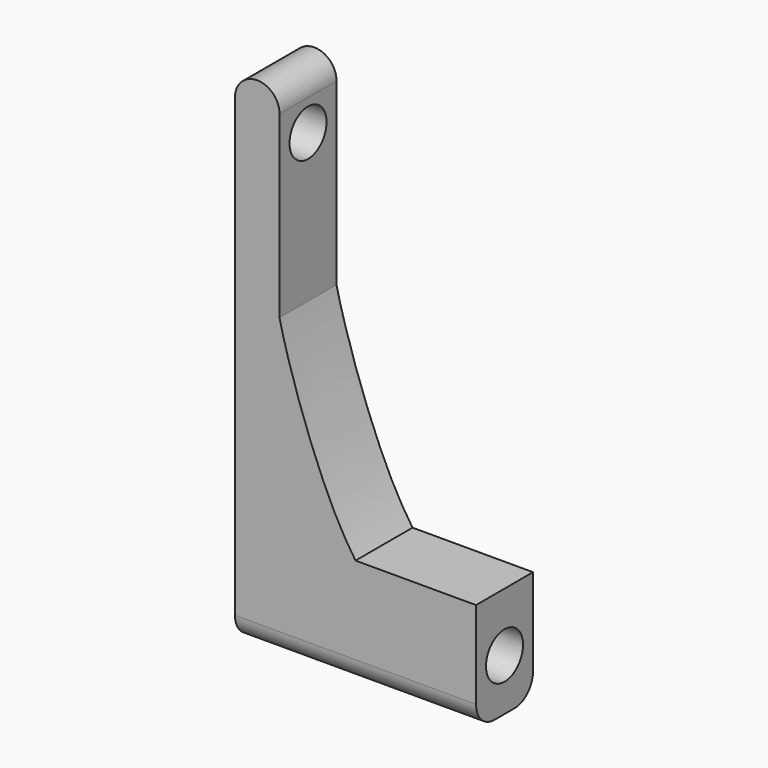
from build123d import *

# Parameters (mm, degrees)
F1_DEPTH = 5.08
F2_R     = 1.651
F4_D     = 3.3


with BuildPart() as f1:
    # F0 (on Front) → F1 (new body)
    with BuildSketch(Plane.XZ):
        with BuildLine():
            Line((-26.6248177087, 44.2240222495), (-26.6248177087, 37.1401777957))
            Line((-26.6248177087, 37.1401777957), (-26.6248177087, 15.790813717))
            Line((-26.6248177087, 15.790813717), (-18.0322819572, 15.790813717))
            Line((-18.0322819572, 15.790813717), (-9.4473101199, 15.790813717))
            Line((-9.4473101199, 15.790813717), (-9.4473101199, 23.6617988805))
            Line((-9.4473101199, 23.6617988805), (-16.3273841628, 23.6617988805))
            add(Edge.make_bspline(
                [(-16.3273841628, 23.6617988805), (-16.2021531976, 23.1573319897), (-16.1372444387, 22.7565283285), (-16.1473177087, 22.4913693964)],
                knots=[0.9536770063, 0.9536770063, 0.9536770063, 0.9536770063, 1, 1, 1, 1], degree=3))
            add(Edge.make_bspline(
                [(-16.1473177087, 22.4913693964), (-16.1800367938, 21.6301041251), (-17.0038324761, 22.1999200382), (-18.0322819572, 23.6617988805)],
                knots=[0, 0, 0, 0, 0.1504621604, 0.1504621604, 0.1504621604, 0.1504621604], degree=3))
            add(Edge.make_bspline(
                [(-18.0322819572, 23.6617988805), (-18.4185584968, 24.2108676593), (-20.6372456091, 27.8178237541), (-22.7930713687, 34.2033705284), (-23.4498177087, 37.1401777957)],
                knots=[0.1504621604, 0.1504621604, 0.1504621604, 0.1504621604, 0.2069744186, 0.4524830891, 0.4524830891, 0.4524830891, 0.4524830891], degree=3))
            add(Edge.make_bspline(
                [(-23.4498177087, 37.1401777957), (-23.7877118735, 38.6511569639), (-23.8355675171, 39.5655078846), (-23.4498177087, 39.3262133002)],
                knots=[0.4524830891, 0.4524830891, 0.4524830891, 0.4524830891, 0.578796617, 0.578796617, 0.578796617, 0.578796617], degree=3))
            Line((-23.4498177087, 39.3262133002), (-23.4498177087, 44.2240222495))
            Line((-23.4498177087, 44.2240222495), (-23.4498177087, 49.9301888049))
            ThreePointArc((-23.4498177087, 49.9301888049), (-25.0373177087, 51.5176888049), (-26.6248177087, 49.9301888049))
            Line((-26.6248177087, 49.9301888049), (-26.6248177087, 44.2240222495))
        make_face()
        with BuildLine():
            Line((-23.4498177087, 37.1401777957), (-23.4498177087, 39.3262133002))
            add(Edge.make_bspline(
                [(-23.4498177087, 37.1401777957), (-23.7877118735, 38.6511569639), (-23.8355675171, 39.5655078846), (-23.4498177087, 39.3262133002)],
                knots=[0.4524830891, 0.4524830891, 0.4524830891, 0.4524830891, 0.578796617, 0.578796617, 0.578796617, 0.578796617], degree=3))
        make_face()
        with BuildLine():
            add(Edge.make_bspline(
                [(-16.3273841628, 23.6617988805), (-16.2021531976, 23.1573319897), (-16.1372444387, 22.7565283285), (-16.1473177087, 22.4913693964)],
                knots=[0.9536770063, 0.9536770063, 0.9536770063, 0.9536770063, 1, 1, 1, 1], degree=3))
            Line((-16.3273841628, 23.6617988805), (-18.0322819572, 23.6617988805))
            add(Edge.make_bspline(
                [(-16.1473177087, 22.4913693964), (-16.1800367938, 21.6301041251), (-17.0038324761, 22.1999200382), (-18.0322819572, 23.6617988805)],
                knots=[0, 0, 0, 0, 0.1504621604, 0.1504621604, 0.1504621604, 0.1504621604], degree=3))
        make_face()
    extrude(amount=F1_DEPTH)

    # F2
    f2_edges = [f1.edges().sort_by_distance(p)[0] for p in [
        (-18.036064, -5.08, 15.790814),
        (-18.036064, 0, 15.790814),
    ]]
    fillet(f2_edges, radius=F2_R)

    # F4 (through all)
    with Locations(Plane(origin=(-26.6248177087, 0, 0), x_dir=(0, -1, 0), z_dir=(-1, 0, 0))):
        with Locations((2.54, 47.7136392146), (2.54, 19.4669695918)):
            Hole(F4_D / 2)


solid = f1.part
